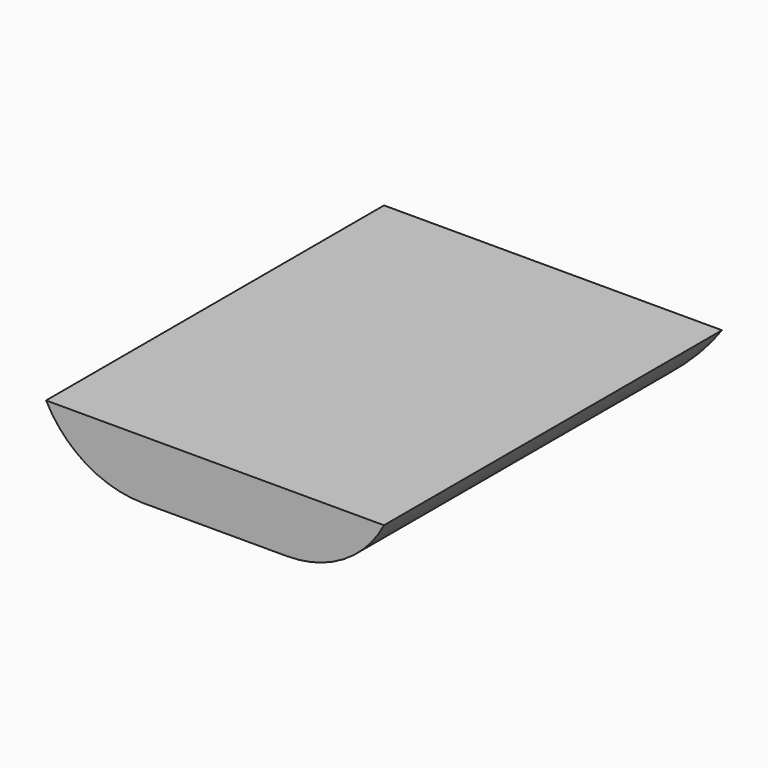
from build123d import *

# Parameters (mm, degrees)
F0_W        = 15.4601242393
F0_H        = 19.3251539022
F1_DEPTH    = 2.68967
F2_T1_DEPTH = 37.6312627369
F2_T3_DEPTH = 41.4962923997


# Not quite as in the source:
# - a fillet or chamfer that OpenCascade refuses, or shapes differently, is made with other operations: its cross-section is extruded or revolved along the edge and cut away or added


with BuildPart() as f1:
    # F0 (on Top) → F1 (new body)
    with BuildSketch(Plane.XY):
        with Locations((-32.5306775048, 23.6733136699)):
            Rectangle(F0_W, F0_H)
    extrude(amount=F1_DEPTH)

    # F2: fillet of radius 5 on 3 edges, made by hand

    # F2_s2 → F2_t1 (cut)
    with BuildSketch(Plane.YZ.offset(-51.3463088733)):
        with BuildLine():
            ThreePointArc((33.3358906209, 2.68967), (31.4947643464, 0.7249766083), (28.9016629214, 0))
            Line((28.9016629214, 0), (33.3358906209, 0))
            Line((33.3358906209, 0), (33.3358906209, 2.68967))
        make_face()
    extrude(amount=F2_T1_DEPTH, mode=Mode.SUBTRACT)

    # F2_s4 → F2_t3 (cut)
    with BuildSketch(Plane.XZ.offset(-44.4214598697)):
        with BuildLine():
            ThreePointArc((-24.8006153852, 2.68967), (-26.6417416597, 0.7249766083), (-29.2348430847, 0))
            Line((-29.2348430847, 0), (-24.8006153852, 0))
            Line((-24.8006153852, 0), (-24.8006153852, 2.68967))
        make_face()
        with BuildLine():
            ThreePointArc((-40.2607396245, 2.68967), (-38.4196133499, 0.7249766083), (-35.826511925, 0))
            Line((-35.826511925, 0), (-40.2607396245, 0))
            Line((-40.2607396245, 0), (-40.2607396245, 2.68967))
        make_face()
    extrude(amount=F2_T3_DEPTH, mode=Mode.SUBTRACT)


solid = f1.part
